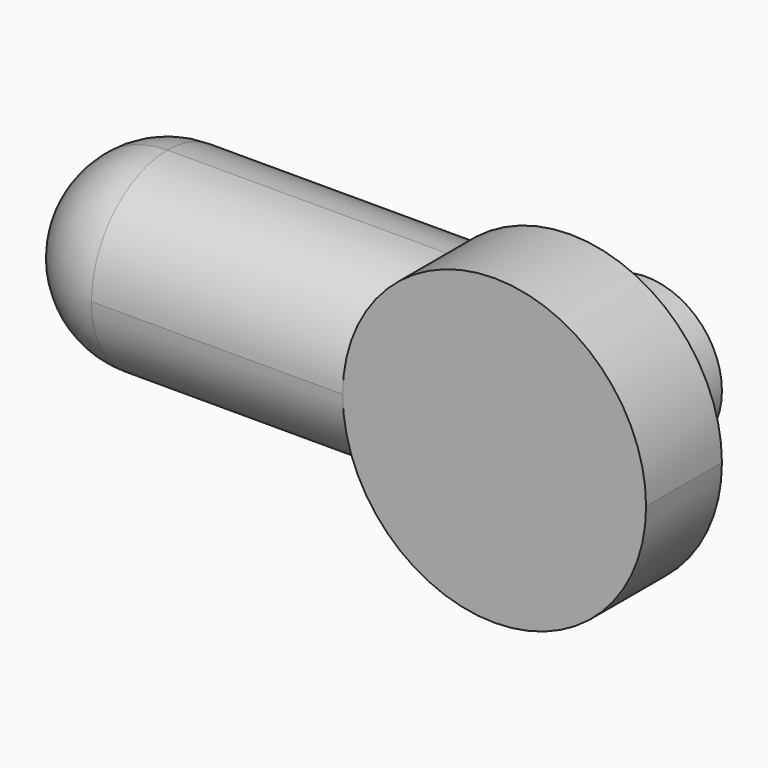
from build123d import *

# Parameters (mm, degrees)
F1_DEPTH = 6.35
F2_R     = 6.3499
F0_R     = 5.08
F3_DEPTH = 6.35
F4_DEPTH = 6.35


# Not quite as in the source:
# - a fillet or chamfer is up to 0.001 mm smaller than in the source, because OpenCascade refuses the exact size


with BuildPart() as f1:
    # F0 (on Front) → F1 (new body, symmetric)
    with BuildSketch(Plane.XZ):
        with BuildLine():
            Line((9.525, 6.35), (-9.525, 6.35))
            Line((-9.525, 6.35), (-9.525, -6.35))
            Line((-9.525, -6.35), (9.525, -6.35))
            ThreePointArc((9.525, -6.35), (7.296147458, 0), (9.525, 6.35))
        make_face()
        with BuildLine():
            Line((-9.525, -6.35), (-9.525, 6.35))
            ThreePointArc((-9.525, 6.35), (-15.875, 0), (-9.525, -6.35))
        make_face()
    extrude(amount=F1_DEPTH, both=True)

    # F2 (radius 6.35 in the source; OpenCascade refuses exactly that, so slightly less here)
    f2_edges = [f1.edges().sort_by_distance(p)[0] for p in [
        (0, -6.35, 6.35),
        (0, 6.35, 6.35),
        (0, -6.35, -6.35),
        (0, 6.35, -6.35),
    ]]
    fillet(f2_edges, radius=F2_R)

    # F0 (on Front) → F3 (join)
    with BuildSketch(Plane.XZ):
        with BuildLine():
            ThreePointArc((27.616147458, 0), (20.8210502669, 9.5866067556), (9.525, 6.35))
            Line((9.525, 6.35), (9.525, -6.35))
            ThreePointArc((9.525, -6.35), (20.8210502669, -9.5866067556), (27.616147458, 0))
        make_face()
        with Locations((17.456147458, 0)):
            Circle(F0_R, mode=Mode.SUBTRACT)
        with BuildLine():
            Line((9.525, -6.35), (9.525, 6.35))
            ThreePointArc((9.525, 6.35), (7.296147458, 0), (9.525, -6.35))
        make_face()
    extrude(amount=F3_DEPTH)

    # F0 (on Front) → F4 (join, symmetric)
    with BuildSketch(Plane.XZ):
        with Locations((17.456147458, 0)):
            Circle(F0_R)
    extrude(amount=F4_DEPTH, both=True)


solid = f1.part
